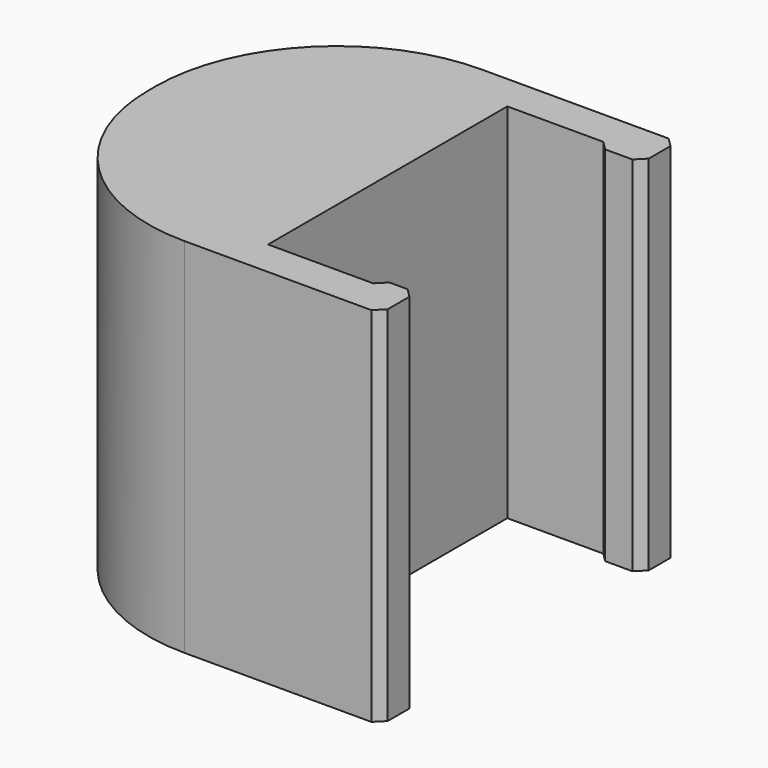
from build123d import *

# Parameters (mm, degrees)
F0_W     = 5.8
F0_H     = 2
F1_DEPTH = 20
F2_R     = 10
F3_SIZE  = 0.49999


# Not quite as in the source:
# - a fillet or chamfer is up to 0.001 mm smaller than in the source, because OpenCascade refuses the exact size


with BuildPart() as f1:
    # F0 (on Top) → F1 (new body)
    with BuildSketch(Plane.XY):
        with Locations((-51.9097009659, 46.350823313)):
            Rectangle(F0_W, F0_H)
        Polygon((-54.8097009659, 45.350823313), (-54.8097009659, 47.350823313), (-67.8097009659, 47.350823313), (-67.8097009659, 26.850823313), (-54.8097009659, 26.850823313), (-54.8097009659, 28.850823313), align=None)
        Polygon((-47.0097009659, 47.350823313), (-49.0097009659, 47.350823313), (-49.0097009659, 45.350823313), (-49.0097009659, 44.850823313), (-47.0097009659, 44.850823313), align=None)
        with Locations((-51.9097009659, 27.850823313)):
            Rectangle(F0_W, F0_H)
        Polygon((-49.0097009659, 29.350823313), (-49.0097009659, 28.850823313), (-49.0097009659, 26.850823313), (-47.0097009659, 26.850823313), (-47.0097009659, 29.350823313), align=None)
    extrude(amount=F1_DEPTH)

    # F2
    f2_edges = [f1.edges().sort_by_distance(p)[0] for p in [
        (-67.809701, 47.350823, 10),
        (-67.809701, 26.850823, 10),
    ]]
    fillet(f2_edges, radius=F2_R)

    # F3 (size 0.5 in the source; OpenCascade refuses exactly that, so slightly less here)
    f3_edges = [f1.edges().sort_by_distance(p)[0] for p in [
        (-47.009701, 47.350823, 10),
        (-47.009701, 44.850823, 10),
        (-47.009701, 29.350823, 10),
        (-47.009701, 26.850823, 10),
        (-49.009701, 29.350823, 10),
        (-49.009701, 45.350823, 10),
    ]]
    chamfer(f3_edges, length=F3_SIZE)


solid = f1.part
